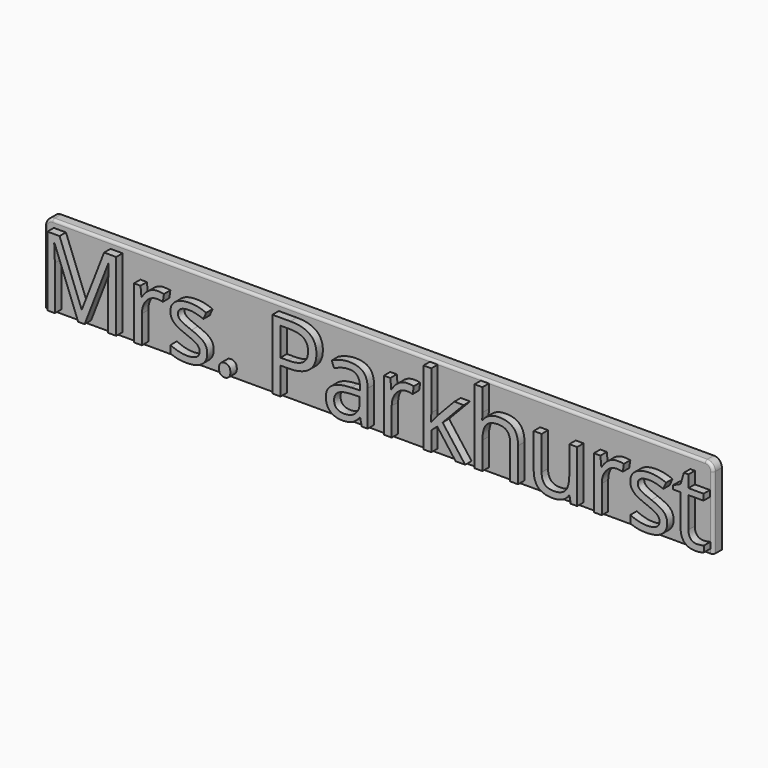
from build123d import *

# Parameters (mm, degrees)
F0_TEXT_SIZE = 36.3521019203
F2_DEPTH     = 3
F1_W         = 250
F1_H         = 30
F3_DEPTH     = 4
F4_R         = 3
F5_R         = 1


# Not quite as in the source:
# - Text() gives the source's letters only with a copy of the font that has no kerning and outlines rounded to 1/6400 em; it was checked with that copy


with BuildPart() as f2:
    # F0 (on Front) → F2 (new body, symmetric)
    with BuildSketch(Plane.XZ):
        with Locations((-120.1745793223, 1.3999999501)):
            Text('Mrs. Parkhurst', F0_TEXT_SIZE, font='Open Sans', text_align=(TextAlign.LEFT, TextAlign.BOTTOM))
    extrude(amount=F2_DEPTH, both=True)


with BuildPart() as f3:
    # F1 (on Front) → F3 (new body)
    with BuildSketch(Plane.XZ):
        with Locations((4.9751272684, 15)):
            Rectangle(F1_W, F1_H)
    extrude(amount=-F3_DEPTH)

    # F4
    f4_edges = [f3.edges().sort_by_distance(p)[0] for p in [
        (-120.024873, 2, 30),
        (129.975127, 2, 30),
    ]]
    fillet(f4_edges, radius=F4_R)

    # F5
    f5_edges = [f3.edges().sort_by_distance(p)[0] for p in [
        (-120.024873, 0, 13.5),
    ]]
    fillet(f5_edges, radius=F5_R)


solid = Compound([f2.part, f3.part])
